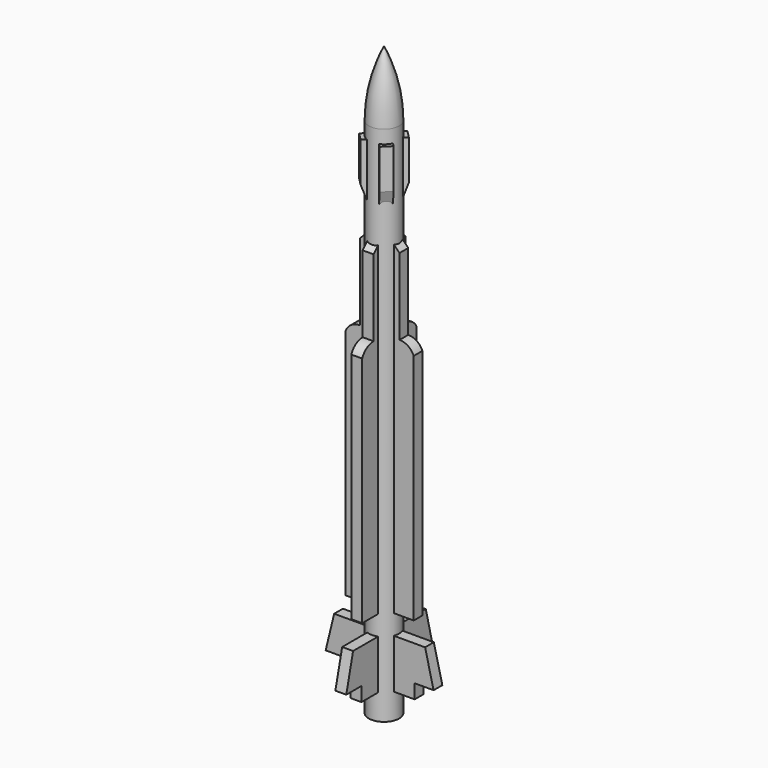
from build123d import *

# Parameters (mm, degrees)
F3_DEPTH     = 0.2
F6_DEPTH     = 0.2
F7_COUNT     = 4
F8_T4_DEPTH  = 1.685841494
F8_S5_R      = 0.5555555556
F8_T6_DEPTH  = 2
F8_T10_DEPTH = 1.685841494
F8_S11_R     = 0.5555555556
F8_T12_DEPTH = 2
F8_T16_DEPTH = 1.685841494
F8_S17_R     = 0.5555555556
F8_T18_DEPTH = 2
F8_T22_DEPTH = 1.685841494
F8_S23_R     = 0.5555555556
F8_T24_DEPTH = 2


# Not quite as in the source:
# - a fillet or chamfer that OpenCascade refuses, or shapes differently, is made with other operations: its cross-section is extruded or revolved along the edge and cut away or added
# - a feature names something its author has since deleted; it is built from what else it names


with BuildPart() as f1:
    # F0 (on Front) → F1 (revolve)
    with BuildSketch(Plane.XZ):
        with BuildLine():
            Line((0, 21.5277777778), (0, 0))
            Line((0, 0), (0.5555555556, 0))
            Line((0.5555555556, 0), (0.5555555556, 19.1319444444))
            ThreePointArc((0.5555555556, 19.1319444444), (0.4148482145, 20.3616455602), (0, 21.5277777778))
        make_face()
    revolve(axis=Axis((0, 0, 10.7638888889), (0, 0, 1)))

    # F2 (on Front) → F3 (join, symmetric)
    with BuildSketch(Plane.XZ):
        with BuildLine():
            Line((0, 15.4166666667), (0, 3.4722222222))
            Line((0, 3.4722222222), (1.25, 3.4722222222))
            Line((1.25, 3.4722222222), (1.25, 12.0138888889))
            ThreePointArc((1.25, 12.0138888889), (1.0421485482, 12.2663478223), (0.7291666667, 12.3611111111))
            Line((0.7291666667, 12.3611111111), (0.7291666667, 15.4166666667))
            Line((0.7291666667, 15.4166666667), (0, 15.4166666667))
        make_face()
        Polygon((0, 2.7430555556), (0, 0.9375), (1.2847222222, 0.9375), (1.2847222222, 1.4583333333), (1.9791666667, 1.4583333333), (1.6666666667, 2.7430555556), align=None)
    extrude(amount=F3_DEPTH, both=True)

    # F5 (on face) → F6 (join, symmetric)
    with BuildSketch(Plane(origin=(0, 0, 0), x_dir=(0.7071067812, -0.7071067812, 0), z_dir=(-0.7071067812, -0.7071067812, 0))):
        Polygon((0, 18.6458333333), (0, 15.2791792114), (0.6944444444, 17.1871496416), (0.6944444444, 18.6458333333), align=None)
    extrude(amount=F6_DEPTH, both=True)

    # F7: F1 ×4 about axis
    f7_axis = Axis((0, 0, 0), (0, 0, 1))


with BuildPart() as f1_1:
    add(f1.part)
    for i in range(1, F7_COUNT):
        add(f1.part.rotate(f7_axis, i * 360 / F7_COUNT))

    # F8: chamfer of 0.25 on 4 edges, made by hand


with BuildPart() as f8_tool2:
    # F8_s3 → F8_t4 (new body)
    with BuildSketch(Plane.XZ.offset(-0.842920747)):
        Polygon((0.7291666667, 15.1666666667), (0.4791666667, 15.4166666667), (0.7291666667, 15.4166666667), align=None)
    extrude(amount=F8_T4_DEPTH)

    # F8_s5 → F8_t6 (cut, symmetric)
    with BuildSketch(Plane.XY.offset(15.3)):
        Circle(F8_S5_R)
    extrude(amount=F8_T6_DEPTH, both=True, mode=Mode.SUBTRACT)


with BuildPart() as f1_2:
    add(f1_1.part)

    # F8_t1: cut F8_tool2
    add(f8_tool2.part, mode=Mode.SUBTRACT)


with BuildPart() as f8_tool8:
    # F8_s9 → F8_t10 (new body)
    with BuildSketch(Plane.YZ.offset(-0.842920747)):
        Polygon((0.7291666667, 15.1666666667), (0.4791666667, 15.4166666667), (0.7291666667, 15.4166666667), align=None)
    extrude(amount=F8_T10_DEPTH)

    # F8_s11 → F8_t12 (cut, symmetric)
    with BuildSketch(Plane.XY.offset(15.3)):
        Circle(F8_S11_R)
    extrude(amount=F8_T12_DEPTH, both=True, mode=Mode.SUBTRACT)


with BuildPart() as f1_3:
    add(f1_2.part)

    # F8_t7: cut F8_tool8
    add(f8_tool8.part, mode=Mode.SUBTRACT)


with BuildPart() as f8_tool14:
    # F8_s15 → F8_t16 (new body)
    with BuildSketch(Plane.XZ.offset(0.842920747)):
        Polygon((-0.7291666667, 15.1666666667), (-0.4791666667, 15.4166666667), (-0.7291666667, 15.4166666667), align=None)
    extrude(amount=-F8_T16_DEPTH)

    # F8_s17 → F8_t18 (cut, symmetric)
    with BuildSketch(Plane.XY.offset(15.3)):
        Circle(F8_S17_R)
    extrude(amount=F8_T18_DEPTH, both=True, mode=Mode.SUBTRACT)


with BuildPart() as f1_4:
    add(f1_3.part)

    # F8_t13: cut F8_tool14
    add(f8_tool14.part, mode=Mode.SUBTRACT)


with BuildPart() as f8_tool20:
    # F8_s21 → F8_t22 (new body)
    with BuildSketch(Plane.YZ.offset(0.842920747)):
        Polygon((-0.7291666667, 15.1666666667), (-0.4791666667, 15.4166666667), (-0.7291666667, 15.4166666667), align=None)
    extrude(amount=-F8_T22_DEPTH)

    # F8_s23 → F8_t24 (cut, symmetric)
    with BuildSketch(Plane.XY.offset(15.3)):
        Circle(F8_S23_R)
    extrude(amount=F8_T24_DEPTH, both=True, mode=Mode.SUBTRACT)


with BuildPart() as f1_5:
    add(f1_4.part)

    # F8_t19: cut F8_tool20
    add(f8_tool20.part, mode=Mode.SUBTRACT)


solid = f1_5.part
